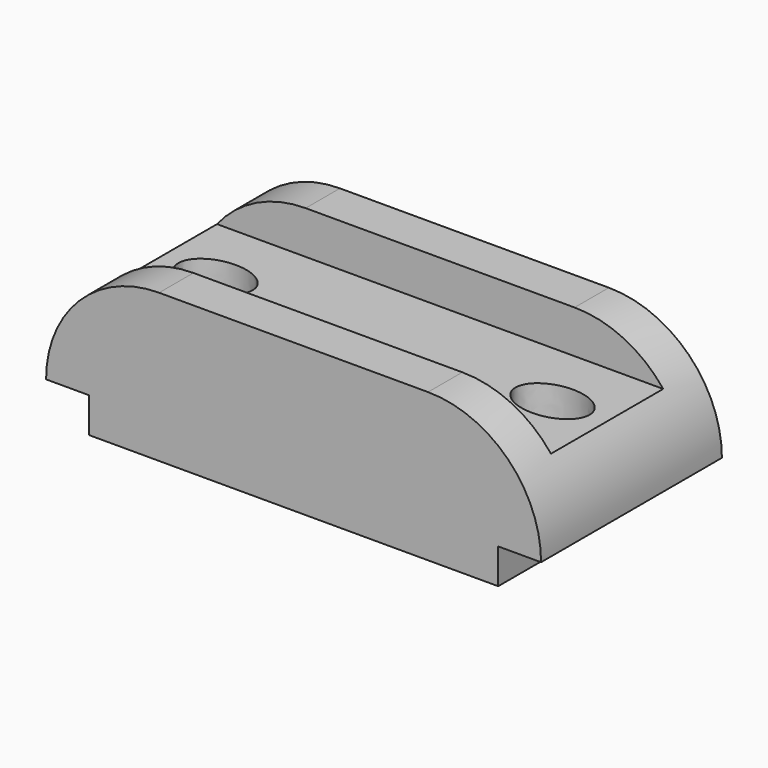
from build123d import *

# Parameters (mm, degrees)
F0_W      = 58
F0_H      = 38
F1_DEPTH  = 127
F2_W      = 58
F2_H      = 9
F3_DEPTH  = 11
F4_W      = 58
F4_H      = 9
F5_DEPTH  = 11
F6_W      = 127
F6_H      = 36
F7_DEPTH  = 11
F8_F1_R   = 28.9999
F8_F2_R   = 28.9999
F12_DEPTH = 38


# Not quite as in the source:
# - a fillet or chamfer is up to 0.001 mm smaller than in the source, because OpenCascade refuses the exact size


with BuildPart() as f1:
    # F0 (on Right) → F1 (new body)
    with BuildSketch(Plane.YZ):
        with Locations((-31.8372100785, 25.0391024165)):
            Rectangle(F0_W, F0_H)
    extrude(amount=F1_DEPTH)

    # F2 (on face) → F3 (cut)
    with BuildSketch(Plane.YZ.offset(127)):
        with Locations((-31.8372100785, 10.5391024165)):
            Rectangle(F2_W, F2_H)
    extrude(amount=-F3_DEPTH, mode=Mode.SUBTRACT)

    # F4 (on face) → F5 (cut)
    with BuildSketch(Plane(origin=(0, 0, 0), x_dir=(0, -1, 0), z_dir=(-1, 0, 0))):
        with Locations((31.8372100785, 10.5391024165)):
            Rectangle(F4_W, F4_H)
    extrude(amount=-F5_DEPTH, mode=Mode.SUBTRACT)

    # F6 (on face) → F7 (cut)
    with BuildSketch(Plane.XY.offset(44.0391024165)):
        with Locations((63.5, -31.8372100785)):
            Rectangle(F6_W, F6_H)
    extrude(amount=-F7_DEPTH, mode=Mode.SUBTRACT)

    # F8: fillet of radius 29 on 4 edges, made by hand

    # F8_f1 (radius 29 in the source; OpenCascade refuses exactly that, so slightly less here)
    f8_f1_edges = [f1.edges().sort_by_distance(p)[0] for p in [
        (0, -8.3372100785, 44.0391024165),
    ]]
    fillet(f8_f1_edges, radius=F8_F1_R)

    # F8_f2 (radius 29 in the source; OpenCascade refuses exactly that, so slightly less here)
    f8_f2_edges = [f1.edges().sort_by_distance(p)[0] for p in [
        (127, -8.3372100785, 44.0391024165),
    ]]
    fillet(f8_f2_edges, radius=F8_F2_R)

    # F11 (on face) → F12 (cut)
    with BuildSketch(Plane.XY.offset(33.0391024165)):
        with BuildLine():
            add(Edge.make_bspline(
                [(29.7623659982, -31.8372100785), (29.7623659982, -20.5788798293), (15.5123659982, -26.2080449539), (1.2623659982, -31.8372100785), (15.5123659982, -37.4663752031), (29.7623659982, -43.0955403277), (29.7623659982, -31.8372100785)],
                knots=[0, 0, 0, 2.0943951024, 2.0943951024, 4.1887902048, 4.1887902048, 6.2831853072, 6.2831853072, 6.2831853072], degree=2, weights=[1, 0.5, 1, 0.5, 1, 0.5, 1]))
        make_face()
        with BuildLine():
            add(Edge.make_bspline(
                [(97.2376340018, -31.8372100785), (97.2376340018, -43.0955403277), (111.4876340018, -37.4663752031), (125.7376340018, -31.8372100785), (111.4876340018, -26.2080449539), (97.2376340018, -20.5788798293), (97.2376340018, -31.8372100785)],
                knots=[0, 0, 0, 2.0943951024, 2.0943951024, 4.1887902048, 4.1887902048, 6.2831853072, 6.2831853072, 6.2831853072], degree=2, weights=[1, 0.5, 1, 0.5, 1, 0.5, 1]))
        make_face()
    extrude(amount=-F12_DEPTH, mode=Mode.SUBTRACT)


solid = f1.part
